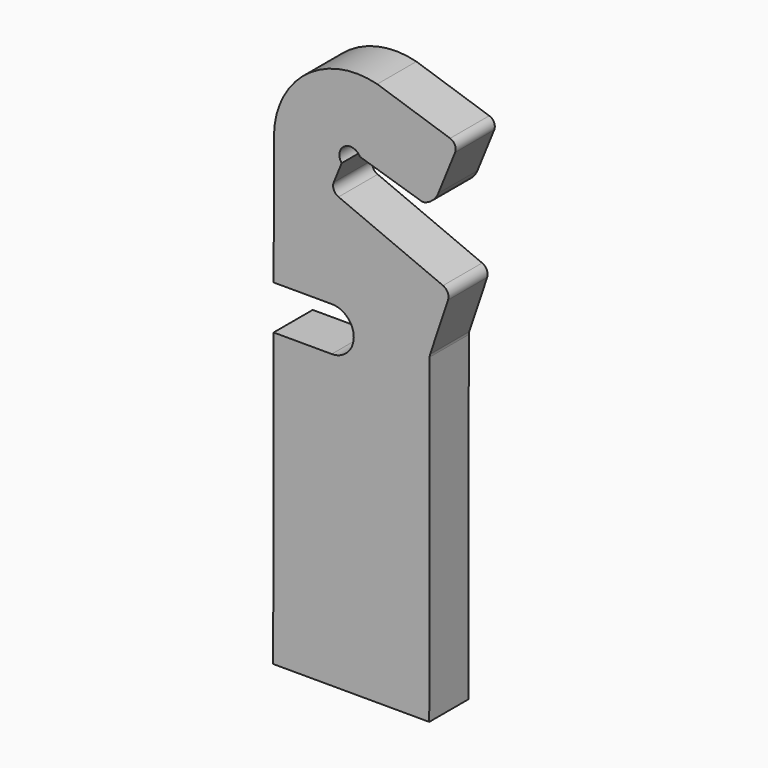
from build123d import *

# Parameters (mm, degrees)
F1_DEPTH = 18
F2_DEPTH = 9


# Not quite as in the source:
# - ends of sketch curves that miss each other by under 0.0002 mm in the source are joined


with BuildPart() as f1:
    # F0 (on Front) → F1 (new body)
    with BuildSketch(Plane.XZ):
        with BuildLine():
            Line((-9.141471, 34.188881), (12.258507, 34.157887))
            ThreePointArc((12.258507, 34.157887), (20.346767, 26.046165), (12.235044, 17.957904))
            Line((12.235044, 17.957904), (-9.164933, 17.988898))
            Line((-9.164933, 17.988898), (-9.294311, -71.341008))
            Line((-9.294311, -71.341008), (9.742649, -71.36858))
            ThreePointArc((9.742649, -71.36858), (12.746991, -68.372928), (15.742643, -71.37727))
            Line((15.742643, -71.37727), (15.729029, -80.77726))
            ThreePointArc((15.729029, -80.77726), (12.724687, -83.772911), (9.729035, -80.76857))
            Line((9.729035, -80.76857), (-9.307925, -80.740999))
            Line((-9.307925, -80.740999), (-9.320635, -89.516989))
            Line((-9.320635, -89.516989), (48.129305, -89.600195))
            Line((48.129305, -89.600195), (48.300632, 28.694563))
            ThreePointArc((48.300632, 28.694563), (48.341618, 29.200469), (48.462079, 29.693531))
            Line((48.462079, 29.693531), (55.053469, 49.381424))
            ThreePointArc((55.053469, 49.381424), (54.931498, 51.787755), (53.20634, 53.469759))
            Line((53.20634, 53.469759), (14.740562, 69.688595))
            ThreePointArc((14.740562, 69.688595), (12.997236, 71.408353), (12.980285, 73.857123))
            Line((12.980285, 73.857123), (15.886835, 81.012644))
            ThreePointArc((15.886835, 81.012644), (16.941219, 86.810977), (22.628344, 85.265342))
            Line((22.628344, 85.265342), (45.010367, 78.329111))
            ThreePointArc((45.010367, 78.329111), (46.013877, 78.196697), (47.004304, 78.405553))
            ThreePointArc((47.004304, 78.405553), (49.689322, 80.161839), (51.468356, 82.83184))
            Line((51.468356, 82.83184), (57.653713, 98.061229))
            ThreePointArc((57.653713, 98.061229), (57.597139, 100.449348), (55.814134, 102.039067))
            Line((55.814134, 102.039067), (28.999419, 110.885722))
            ThreePointArc((28.999419, 110.885722), (2.856816, 105.590311), (-9.035869, 81.714778))
            Line((-9.035869, 81.714778), (-9.141471, 34.188881))
        make_face()
        with BuildLine():
            ThreePointArc((39.177572, -56.266483), (42.347971, -59.446078), (39.168375, -62.616476))
            Line((39.168375, -62.616476), (30.168385, -62.603441))
            ThreePointArc((30.168385, -62.603441), (26.997987, -59.423846), (30.177582, -56.253447))
            Line((30.177582, -56.253447), (30.304019, 31.046461))
            ThreePointArc((30.304019, 31.046461), (27.133621, 34.226056), (30.313216, 37.396454))
            Line((30.313216, 37.396454), (39.313207, 37.383419))
            ThreePointArc((39.313207, 37.383419), (42.483605, 34.203824), (39.30401, 31.033426))
            Line((39.30401, 31.033426), (39.177572, -56.266483))
        make_face(mode=Mode.SUBTRACT)
        with BuildLine():
            Line((30.168385, -62.603441), (39.168375, -62.616476))
            ThreePointArc((39.168375, -62.616476), (42.347971, -59.446078), (39.177572, -56.266483))
            Line((39.177572, -56.266483), (39.30401, 31.033426))
            ThreePointArc((39.30401, 31.033426), (42.483605, 34.203824), (39.313207, 37.383419))
            Line((39.313207, 37.383419), (30.313216, 37.396454))
            ThreePointArc((30.313216, 37.396454), (27.133621, 34.226056), (30.304019, 31.046461))
            Line((30.304019, 31.046461), (30.177582, -56.253448))
            ThreePointArc((30.177582, -56.253448), (26.997987, -59.423846), (30.168385, -62.603441))
        make_face()
        with BuildLine():
            Line((9.742649, -71.36858), (-9.294311, -71.341008))
            Line((-9.294311, -71.341008), (-9.307925, -80.740999))
            Line((-9.307925, -80.740999), (9.729035, -80.76857))
            ThreePointArc((9.729035, -80.76857), (12.724687, -83.772911), (15.729029, -80.77726))
            Line((15.729029, -80.77726), (15.742643, -71.37727))
            ThreePointArc((15.742643, -71.37727), (12.746991, -68.372928), (9.742649, -71.36858))
        make_face()
    extrude(amount=F1_DEPTH)

    # F0 (on Front) → F2 (cut)
    with BuildSketch(Plane.XZ):
        with BuildLine():
            Line((9.742649, -71.36858), (-9.294311, -71.341008))
            Line((-9.294311, -71.341008), (-9.307925, -80.740999))
            Line((-9.307925, -80.740999), (9.729035, -80.76857))
            ThreePointArc((9.729035, -80.76857), (12.724687, -83.772911), (15.729029, -80.77726))
            Line((15.729029, -80.77726), (15.742643, -71.37727))
            ThreePointArc((15.742643, -71.37727), (12.746991, -68.372928), (9.742649, -71.36858))
        make_face()
        with BuildLine():
            Line((30.168385, -62.603441), (39.168375, -62.616476))
            ThreePointArc((39.168375, -62.616476), (42.347971, -59.446078), (39.177572, -56.266483))
            Line((39.177572, -56.266483), (39.30401, 31.033426))
            ThreePointArc((39.30401, 31.033426), (42.483605, 34.203824), (39.313207, 37.383419))
            Line((39.313207, 37.383419), (30.313216, 37.396454))
            ThreePointArc((30.313216, 37.396454), (27.133621, 34.226056), (30.304019, 31.046461))
            Line((30.304019, 31.046461), (30.177582, -56.253448))
            ThreePointArc((30.177582, -56.253448), (26.997987, -59.423846), (30.168385, -62.603441))
        make_face()
    extrude(amount=F2_DEPTH, mode=Mode.SUBTRACT)


solid = f1.part
